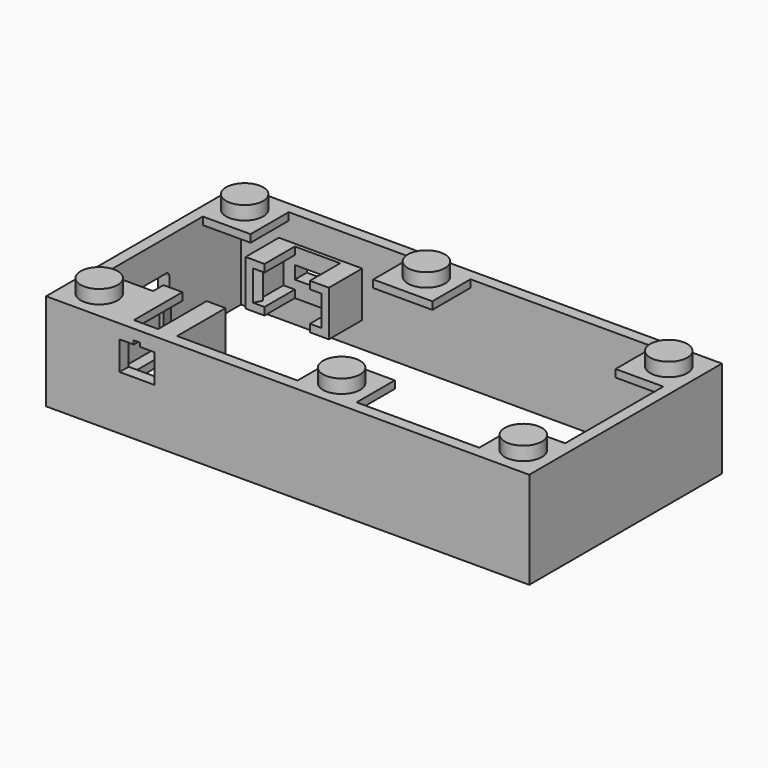
from build123d import *

# Parameters (mm, degrees)
F0_W      = 63.8
F0_H      = 31.8
F0_W_2    = 60.8
F0_H_2    = 28.8
F1_DEPTH  = 12.8
F2_W      = 6.3
F2_H      = 6.3
F2_W_2    = 7.8
F3_DEPTH  = 1
F4_R      = 2.45
F5_DEPTH  = 1.8
F6_W      = 0.85
F6_H      = 0.5
F7_DEPTH  = 25.4
F9_DEPTH  = 8
F11_DEPTH = 5
F12_W     = 0.1
F12_H     = 1
F13_DEPTH = 6.3
F14_W     = 6
F14_H     = 1.7
F15_DEPTH = 2.54
F16_W     = 11
F16_H     = 6
F16_W_2   = 6
F16_H_2   = 1.7
F17_DEPTH = 0.5
F19_DEPTH = 5
F21_DEPTH = 4
F23_DEPTH = 25.4


# Not quite as in the source:
# - a feature names something its author has since deleted; it is built from what else it names


with BuildPart() as f1:
    # F0 (on Top) → F1 (new body)
    with BuildSketch(Plane.XY):
        with Locations((31.9, 15.9)):
            Rectangle(F0_W, F0_H)
        with Locations((31.9, 15.9)):
            Rectangle(F0_W_2, F0_H_2, mode=Mode.SUBTRACT)
    extrude(amount=F1_DEPTH)

    # F2 (on face) → F3 (join)
    with BuildSketch(Plane.XY.offset(12.8)):
        with Locations((4.65, 27.15)):
            Rectangle(F2_W, F2_H)
        with Locations((4.65, 4.65)):
            Rectangle(F2_W, F2_H)
        with Locations((59.15, 4.65)):
            Rectangle(F2_W, F2_H)
        with Locations((59.15, 27.15)):
            Rectangle(F2_W, F2_H)
        with Locations((27.9, 27.15)):
            Rectangle(F2_W_2, F2_H)
        with Locations((35.9, 4.65)):
            Rectangle(F2_W_2, F2_H)
    extrude(amount=-F3_DEPTH)

    # F4 (on face) → F5 (join)
    with BuildSketch(Plane.XY.offset(12.8)):
        with Locations((3.9, 27.9)):
            Circle(F4_R)
        with Locations((59.9, 27.9)):
            Circle(F4_R)
        with Locations((59.9, 3.9)):
            Circle(F4_R)
        with Locations((3.9, 3.9)):
            Circle(F4_R)
        with Locations((27.9, 27.9)):
            Circle(F4_R)
        with Locations((35.9, 3.9)):
            Circle(F4_R)
    extrude(amount=F5_DEPTH)

    # F6 (on face) → F7 (cut)
    with BuildSketch(Plane.XZ):
        Polygon((11.575, 10.95), (9.7, 10.95), (9.7, 7.15), (14.3, 7.15), (14.3, 10.95), (12.425, 10.95), align=None)
        with Locations((12, 11.2)):
            Rectangle(F6_W, F6_H)
    extrude(amount=-F7_DEPTH, mode=Mode.SUBTRACT)

    # F8 (on face) → F9 (join)
    with BuildSketch(Plane(origin=(0, 1.5, 0), x_dir=(-1, 0, 0), z_dir=(0, 1, 0))):
        Polygon((-13.6, 5.8), (-13.6, 6.8), (-15.1, 6.8), (-15.1, 11.8), (-13.6, 11.8), (-13.6, 12.8), (-16.1, 12.8), (-16.1, 5.8), align=None)
        Polygon((-8.9, 6.8), (-10.4, 6.8), (-10.4, 5.8), (-7.9, 5.8), (-7.9, 12.8), (-10.4, 12.8), (-10.4, 11.8), (-8.9, 11.8), align=None)
    extrude(amount=F9_DEPTH)

    # F10 (on face) → F11 (join, through all)
    with BuildSketch(Plane.XY.offset(6.8)):
        Polygon((14.6, 7.6), (15.1, 7.6), (15.1, 9.5), align=None)
        Polygon((9.4, 7.6), (8.9, 9.5), (8.9, 7.6), align=None)
    extrude(amount=F11_DEPTH)

    # F12 (on face) → F13 (join, through all)
    with BuildSketch(Plane(origin=(0, 1.5, 0), x_dir=(-1, 0, 0), z_dir=(0, 1, 0))):
        with Locations((-7.85, 12.3)):
            Rectangle(F12_W, F12_H)
    extrude(amount=F13_DEPTH)

    # F14 (on face) → F15 (cut)
    with BuildSketch(Plane(origin=(0, 31.8, 0), x_dir=(-1, 0, 0), z_dir=(0, 1, 0))):
        with Locations((-12, 6.4)):
            Rectangle(F14_W, F14_H)
    extrude(amount=-F15_DEPTH, mode=Mode.SUBTRACT)

    # F16 (on face) → F17 (join)
    with BuildSketch(Plane.XZ.offset(-30.3)):
        with Locations((12, 6.4)):
            Rectangle(F16_W, F16_H)
        with Locations((12, 6.4)):
            Rectangle(F16_W_2, F16_H_2, mode=Mode.SUBTRACT)
    extrude(amount=F17_DEPTH)

    # F18 (on face) → F19 (join)
    with BuildSketch(Plane.XZ.offset(-29.8)):
        Polygon((9, 9.4), (6.5, 9.4), (6.5, 3.4), (9, 3.4), (9, 4.4), (7.5, 4.4), (7.5, 8.4), (9, 8.4), align=None)
        Polygon((17.5, 9.4), (15, 9.4), (15, 8.4), (16.5, 8.4), (16.5, 4.4), (15, 4.4), (15, 3.4), (17.5, 3.4), align=None)
    extrude(amount=F19_DEPTH)

    # F20 (on face) → F21 (join, through all)
    with BuildSketch(Plane.XY.offset(4.4)):
        Polygon((7.5, 25.8), (7.5, 24.8), (8, 25.8), align=None)
        Polygon((16, 25.8), (16.5, 24.8), (16.5, 25.8), align=None)
    extrude(amount=F21_DEPTH)

    # F22 (on face) → F23 (cut)
    with BuildSketch(Plane(origin=(0, 0, 0), x_dir=(0, -1, 0), z_dir=(-1, 0, 0))):
        with BuildLine():
            Line((-13.8921684574, 8.65), (-17.9078315426, 8.65))
            ThreePointArc((-17.9078315426, 8.65), (-18.3088802049, 8.4838802049), (-18.475, 8.0828315426))
            Line((-18.475, 8.0828315426), (-18.475, 4.7171684574))
            ThreePointArc((-18.475, 4.7171684574), (-18.3088802049, 4.3161197951), (-17.9078315426, 4.15))
            Line((-17.9078315426, 4.15), (-13.8921684574, 4.15))
            ThreePointArc((-13.8921684574, 4.15), (-13.4911197951, 4.3161197951), (-13.325, 4.7171684574))
            Line((-13.325, 4.7171684574), (-13.325, 8.0828315426))
            ThreePointArc((-13.325, 8.0828315426), (-13.4911197951, 8.4838802049), (-13.8921684574, 8.65))
        make_face()
    extrude(amount=-F23_DEPTH, mode=Mode.SUBTRACT)


solid = f1.part
